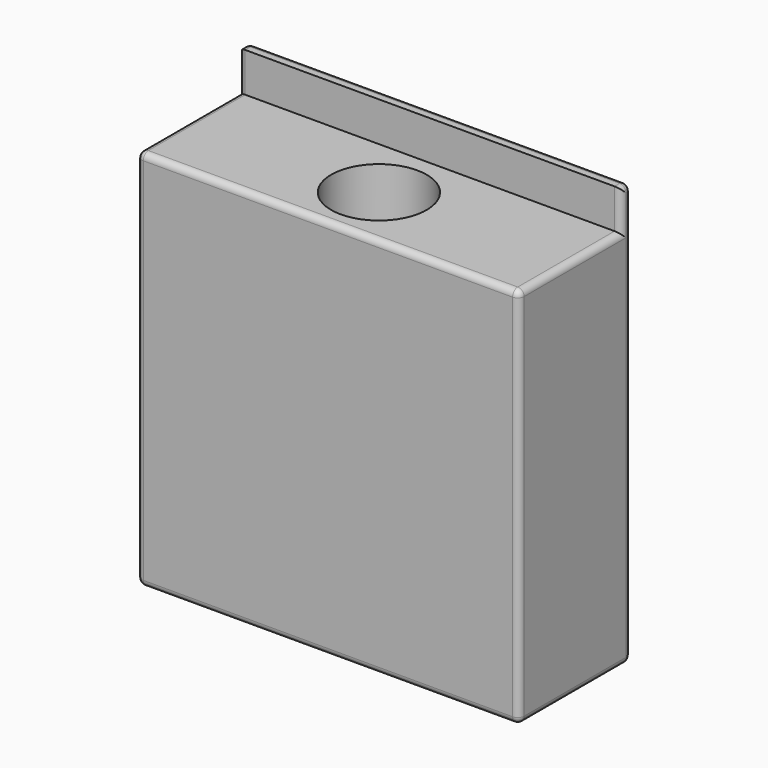
from build123d import *

# Parameters (mm, degrees)
F1_DEPTH = 60
F3_DEPTH = 60
F4_R     = 0.99999


# Not quite as in the source:
# - a fillet or chamfer is up to 0.001 mm smaller than in the source, because OpenCascade refuses the exact size
# - the program builds the solid bodies; features that only make, move or delete a surface that nothing else refers to are left out


with BuildPart() as f1:
    # F0 (on Top) → F1 (new body)
    with BuildSketch(Plane.XY):
        with BuildLine():
            Line((-60, 20), (-60, 10))
            Line((-60, 10), (-37.5, 10))
            ThreePointArc((-37.5, 10), (-35.3033008589, 15.3033008589), (-30, 17.5))
            Line((-30, 17.5), (-30, 20))
            Line((-30, 20), (-60, 20))
        make_face()
        with BuildLine():
            Line((-22.5, 10), (0, 10))
            Line((0, 10), (0, 20))
            Line((0, 20), (-30, 20))
            Line((-30, 20), (-30, 17.5))
            ThreePointArc((-30, 17.5), (-24.6966991411, 15.3033008589), (-22.5, 10))
        make_face()
        with BuildLine():
            Line((-30, 0), (0, 0))
            Line((0, 0), (0, 10))
            Line((0, 10), (-22.5, 10))
            ThreePointArc((-22.5, 10), (-24.6966991411, 4.6966991411), (-30, 2.5))
            Line((-30, 2.5), (-30, 0))
        make_face()
        with BuildLine():
            Line((-60, 0), (-30, 0))
            Line((-30, 0), (-30, 2.5))
            ThreePointArc((-30, 2.5), (-35.3033008589, 4.6966991411), (-37.5, 10))
            Line((-37.5, 10), (-60, 10))
            Line((-60, 10), (-60, 0))
        make_face()
    extrude(amount=F1_DEPTH)

    # F2 (on face) → F3 (join)
    with BuildSketch(Plane(origin=(-60, 0, 0), x_dir=(0, -1, 0), z_dir=(-1, 0, 0))):
        Polygon((-22, 0), (-20, 0), (-20, 60), (-20, 66.1894296401), (-22, 66.1894296401), align=None)
    extrude(amount=-F3_DEPTH)

    # F4 (radius 1 in the source; OpenCascade refuses exactly that, so slightly less here)
    f4_edges = [f1.edges().sort_by_distance(p)[0] for p in [
        (0, 22, 33.094715),
        (-60, 0, 30),
        (-60, 11, 0),
        (-60, 22, 33.094715),
        (-60, 21, 66.18943),
        (-60, 20, 63.094715),
        (-60, 10, 60),
        (-30, 22, 66.18943),
        (-30, 22, 0),
        (-30, 0, 0),
        (0, 11, 0),
        (-30, 17.5, 0),
        (0, 0, 30),
        (0, 10, 60),
        (0, 20, 63.094715),
        (0, 21, 66.18943),
        (-30, 0, 60),
    ]]
    fillet(f4_edges, radius=F4_R)


solid = f1.part
